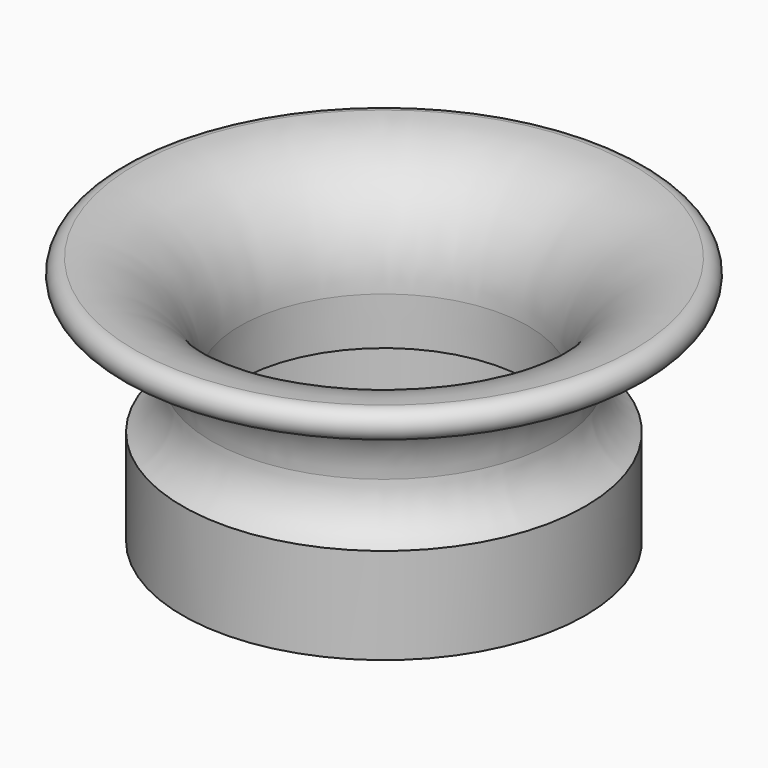
from build123d import *


# Not quite as in the source:
# - a feature of the source that left no trace in its solid (it failed there, or was rolled back) is left out
# - a feature names something its author has since deleted; it is built from what else it names


with BuildPart() as f1:
    # F0 (on Front) → F1 (revolve)
    with BuildSketch(Plane.XZ):
        with BuildLine():
            ThreePointArc((10.9666396311, 27.1683829889), (12.4701625396, 28.6523491091), (10.9666396311, 30.1363152292))
            ThreePointArc((10.9666396311, 30.1363152292), (3.1518347441, 26.8641196143), (0, 19))
            Line((0, 19), (0.0767615013, 14.0005892675))
            Line((0.0767615013, 14.0005892675), (2.9666396311, 14.0449607736))
            Line((2.9666396311, 14.0449607736), (2.9666396311, 4.1683829889))
            Line((2.9666396311, 4.1683829889), (5.9666396311, 4.1683829889))
            Line((5.9666396311, 4.1683829889), (5.9666396311, 14.1683829889))
            ThreePointArc((5.9666396311, 14.1683829889), (3.7741797187, 16.2529070415), (2.9666396311, 19.1683829889))
            ThreePointArc((2.9666396311, 19.1683829889), (5.3097853816, 24.8252372384), (10.9666396311, 27.1683829889))
        make_face()
    revolve(axis=Axis((-15, 0, 28.4551028162), (0, 0, 1)))


solid = f1.part
